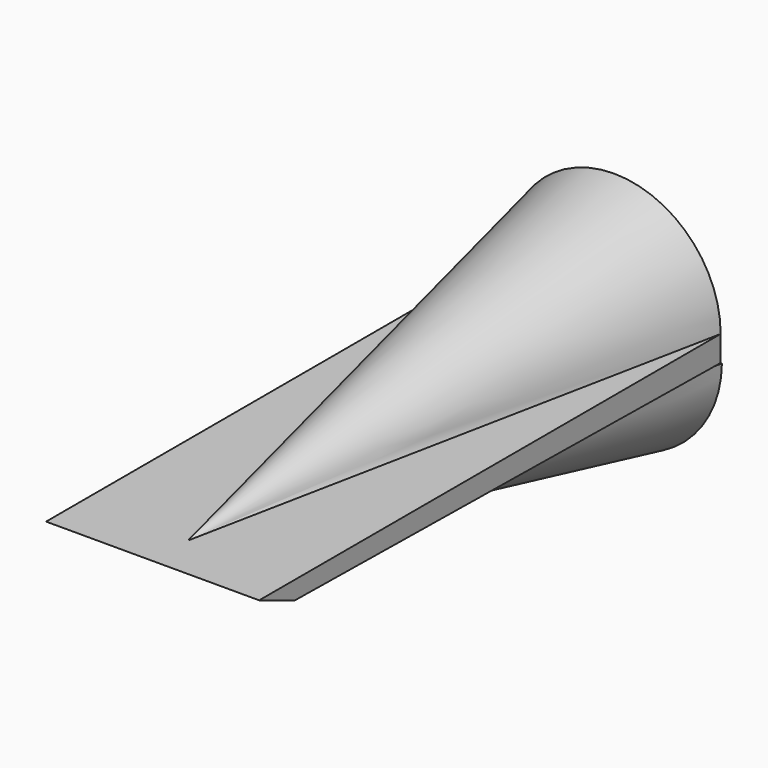
from build123d import *

# Parameters (mm, degrees)
F1_ANGLE_BACK = 90
F1_ANGLE      = 180
F3_ANGLE_BACK = 90
F3_ANGLE      = 180
F5_DEPTH      = 20
F6_DEPTH      = 20


with BuildPart() as f1:
    # F0 (on Right) → F1 (revolve)
    with BuildSketch(Plane.YZ, mode=Mode.PRIVATE) as f1_sk:
        Polygon((-100, 0), (0, 0), (0, 20), align=None)
    revolve(f1_sk.sketch.rotate(Axis((0, -50, 0), (0, -1, 0)), -F1_ANGLE_BACK), axis=Axis((0, -50, 0), (0, -1, 0)), revolution_arc=F1_ANGLE)

    # F4 (on Right) → F5 (join)
    with BuildSketch(Plane.YZ):
        Polygon((0, -4.7873738222), (0, 0), (-99.9898836017, 0), (-108.3033829927, 0), (-99.9898836017, -3.4161338117), align=None)
    extrude(amount=F5_DEPTH)

    # F4 (on Right) → F6 (join)
    with BuildSketch(Plane.YZ):
        Polygon((0, -4.7873738222), (0, 0), (-99.9898836017, 0), (-108.3033829927, 0), (-99.9898836017, -3.4161338117), align=None)
    extrude(amount=-F6_DEPTH)


with BuildPart() as f3:
    # F2 (on Right) → F3 (revolve)
    with BuildSketch(Plane.YZ, mode=Mode.PRIVATE) as f3_sk:
        Polygon((0, -25), (0, -5), (-99.988911184, -3.510825649), align=None)
    revolve(f3_sk.sketch.rotate(Axis((0, -49.994455592, -4.2554128245), (0, 0.9998891118, -0.0148917435)), -F3_ANGLE_BACK), axis=Axis((0, -49.994455592, -4.2554128245), (0, 0.9998891118, -0.0148917435)), revolution_arc=F3_ANGLE)


solid = Compound([f1.part, f3.part])
